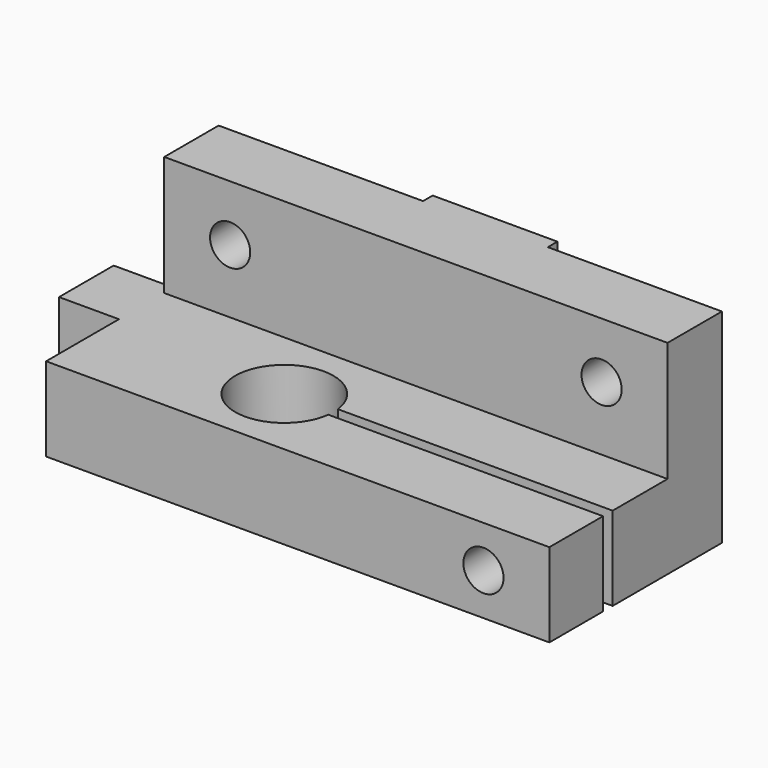
from build123d import *

# Parameters (mm, degrees)
F0_W          = 42
F0_H          = 18
F1_DEPTH      = 7
F4_DEPTH      = 25
F5_W          = 42
F5_H          = 5.6745335534
F6_DEPTH      = 10
F7_R          = 1.675
F8_DEPTH      = 25
F9_DEPTH      = 25
F10_TEXT_SIZE = 23.6111111111
F11_DEPTH     = 1
F12_W         = 5.7
F12_H         = 7
F13_DEPTH     = 5


# Not quite as in the source:
# - Text() gives the source's letters only with a copy of the font that has no kerning and outlines rounded to 1/6400 em; it was checked with that copy


with BuildPart() as f1:
    # F0 (on Top) → F1 (new body)
    with BuildSketch(Plane.XY):
        with Locations((21, 9)):
            Rectangle(F0_W, F0_H)
    extrude(amount=F1_DEPTH)

    # F3 (on face) → F4 (cut)
    with BuildSketch(Plane(origin=(0, 18, 0), x_dir=(-1, 0, 0), z_dir=(0, 1, 0))):
        with BuildLine():
            ThreePointArc((-38.175, 3.5), (-36.5, 1.825), (-34.825, 3.5))
            ThreePointArc((-34.825, 3.5), (-36.5, 5.175), (-38.175, 3.5))
        make_face()
    extrude(amount=-F4_DEPTH, mode=Mode.SUBTRACT)

    # F5 (on face) → F6 (join)
    with BuildSketch(Plane.XY.offset(7)):
        with Locations((21, 15.1627332233)):
            Rectangle(F5_W, F5_H)
    extrude(amount=F6_DEPTH)

    # F7 (on face) → F8 (cut)
    with BuildSketch(Plane(origin=(0, 18, 0), x_dir=(-1, 0, 0), z_dir=(0, 1, 0))):
        with Locations((-36.5, 12.325)):
            Circle(F7_R)
        with Locations((-5.5, 12.325)):
            Circle(F7_R)
    extrude(amount=-F8_DEPTH, mode=Mode.SUBTRACT)

    # F2 (on face) → F9 (cut)
    with BuildSketch(Plane.XY.offset(7)):
        with BuildLine():
            ThreePointArc((19.0693979899, 5.6), (19.0923423463, 5.8495321962), (19.1, 6.1))
            ThreePointArc((19.1, 6.1), (19.0923423463, 6.3504678038), (19.0693979899, 6.6))
            ThreePointArc((19.0693979899, 6.6), (10.9, 6.1), (19.0693979899, 5.6))
        make_face()
        with BuildLine():
            Line((42, 6.1), (19.1, 6.1))
            ThreePointArc((19.1, 6.1), (19.0923423463, 5.8495321962), (19.0693979899, 5.6))
            Line((19.0693979899, 5.6), (42, 5.6))
            Line((42, 5.6), (42, 6.1))
        make_face()
        with BuildLine():
            ThreePointArc((19.0693979899, 6.6), (19.0923423463, 6.3504678038), (19.1, 6.1))
            Line((19.1, 6.1), (42, 6.1))
            Line((42, 6.1), (42, 6.6))
            Line((42, 6.6), (19.0693979899, 6.6))
        make_face()
    extrude(amount=-F9_DEPTH, mode=Mode.SUBTRACT)

    # F10 (on face) → F11 (join)
    with BuildSketch(Plane(origin=(0, 18, 0), x_dir=(-1, 0, 0), z_dir=(0, 1, 0))):
        with Locations(Location((-14.9393391335, 17), (0, 0, -180))):
            Text('L', F10_TEXT_SIZE, font='Open Sans', font_style=FontStyle.BOLD, text_align=(TextAlign.LEFT, TextAlign.BOTTOM))
    extrude(amount=F11_DEPTH)

    # F12 (on face) → F13 (join)
    with BuildSketch(Plane(origin=(0, 0, 0), x_dir=(0, -1, 0), z_dir=(-1, 0, 0))):
        with Locations((-10.45, 3.5)):
            Rectangle(F12_W, F12_H)
    extrude(amount=F13_DEPTH)


solid = f1.part
